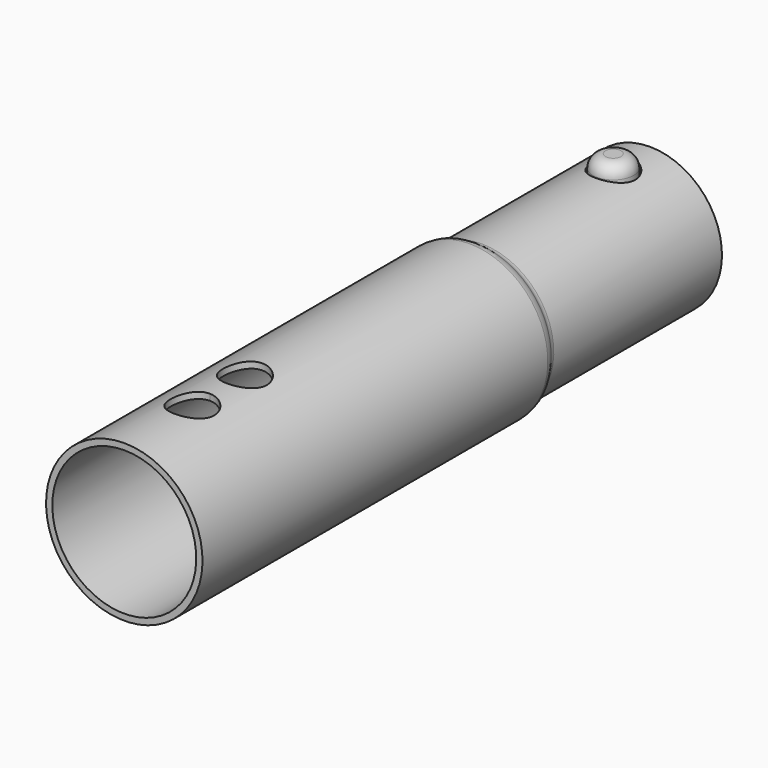
from build123d import *

# Parameters (mm, degrees)
F2_T     = -1
F4_R     = 2
F6_DEPTH = 15
F8_R     = 3.25
F9_DEPTH = 7.5
F10_R    = 2


# Not quite as in the source:
# - a fillet or chamfer that OpenCascade refuses, or shapes differently, is made with other operations: its cross-section is extruded or revolved along the edge and cut away or added
# - a feature names something its author has since deleted; it is built from what else it names


with BuildPart() as f1:
    # F0 (on Right) → F1 (revolve)
    with BuildSketch(Plane.YZ):
        Polygon((-61.0685050488, 12.5), (-61.0685050488, 0), (43.9314949512, 0), (43.9314949512, 11.5), (8.9314949512, 11.5), (8.9314949512, 12.5), align=None)
    revolve(axis=Axis((0, -8.5685050488, 0), (0, -1, 0)))

    # F2
    f2_openings = [f1.faces().sort_by_distance(p)[0] for p in [
        (0, -61.068505, 0),
        (0, 43.931495, 0),
    ]]
    offset(amount=F2_T, openings=f2_openings, kind=Kind.INTERSECTION)

    # F3: fillet of radius 1.5 on 1 edges, made by hand

    # F3_s1 → F3_t2 (revolve)
    with BuildSketch(Plane.YZ):
        with BuildLine():
            ThreePointArc((10.3457085136, 11.5), (9.4796831098, 11.7752551286), (8.9314949512, 12.5))
            Line((8.9314949512, 12.5), (8.9314949512, 11.5))
            Line((8.9314949512, 11.5), (10.3457085136, 11.5))
        make_face()
    revolve(axis=Axis((0, 8.9314949512, 0), (0, -1, 0)))

    # F4
    f4_edges = [f1.edges().sort_by_distance(p)[0] for p in [
        (0, 8.931495, -12.5),
    ]]
    fillet(f4_edges, radius=F4_R)

    # F5 (on Top) → F6 (cut)
    with BuildSketch(Plane.XY):
        with BuildLine():
            ThreePointArc((3.5, -36.9775111079), (-2.4748737342, -34.5026373738), (0, -40.4775111079))
            ThreePointArc((0, -40.4775111079), (2.4748737342, -39.4523848421), (3.5, -36.9775111079))
        make_face()
        with BuildLine():
            ThreePointArc((3.25, -36.9775111079), (2.2980970389, -39.2756081468), (0, -40.2275111079))
            ThreePointArc((0, -40.2275111079), (-2.2980970389, -34.6794140691), (3.25, -36.9775111079))
        make_face(mode=Mode.SUBTRACT)
        with BuildLine():
            ThreePointArc((3.5, 36.6118407249), (2.4748737342, 39.0867144591), (0, 40.1118407249))
            ThreePointArc((0, 40.1118407249), (-2.4748737342, 34.1369669908), (3.5, 36.6118407249))
        make_face()
        with BuildLine():
            ThreePointArc((3.25, 36.6118407249), (-2.2980970389, 34.3137436861), (0, 39.8618407249))
            ThreePointArc((0, 39.8618407249), (2.2980970389, 38.9099377638), (3.25, 36.6118407249))
        make_face(mode=Mode.SUBTRACT)
        with BuildLine():
            ThreePointArc((3.25, 36.6118407249), (2.2980970389, 38.9099377638), (0, 39.8618407249))
            ThreePointArc((0, 39.8618407249), (-2.2980970389, 34.3137436861), (3.25, 36.6118407249))
        make_face()
        with BuildLine():
            ThreePointArc((3.25, -36.9775111079), (-2.2980970389, -34.6794140691), (0, -40.2275111079))
            ThreePointArc((0, -40.2275111079), (2.2980970389, -39.2756081468), (3.25, -36.9775111079))
        make_face()
        with BuildLine():
            Line((0, -43.9788174033), (0, -50.9788174033))
            ThreePointArc((0, -50.9788174033), (2.4748737342, -49.9536911375), (3.5, -47.4788174033))
            ThreePointArc((3.5, -47.4788174033), (2.4748737342, -45.0039436692), (0, -43.9788174033))
        make_face()
        with BuildLine():
            ThreePointArc((0, -43.9788174033), (-3.5, -47.4788174033), (0, -50.9788174033))
            Line((0, -50.9788174033), (0, -43.9788174033))
        make_face()
    extrude(amount=F6_DEPTH, mode=Mode.SUBTRACT)


with BuildPart() as f9:
    # F8 (on offset) → F9 (new body)
    with BuildSketch(Plane.XY.offset(6)):
        with Locations((0, 36.5961231291)):
            Circle(F8_R)
    extrude(amount=F9_DEPTH)

    # F10
    f10_edges = [f9.edges().sort_by_distance(p)[0] for p in [
        (-3.25, 36.596123, 13.5),
    ]]
    fillet(f10_edges, radius=F10_R)


solid = Compound([f1.part, f9.part])
